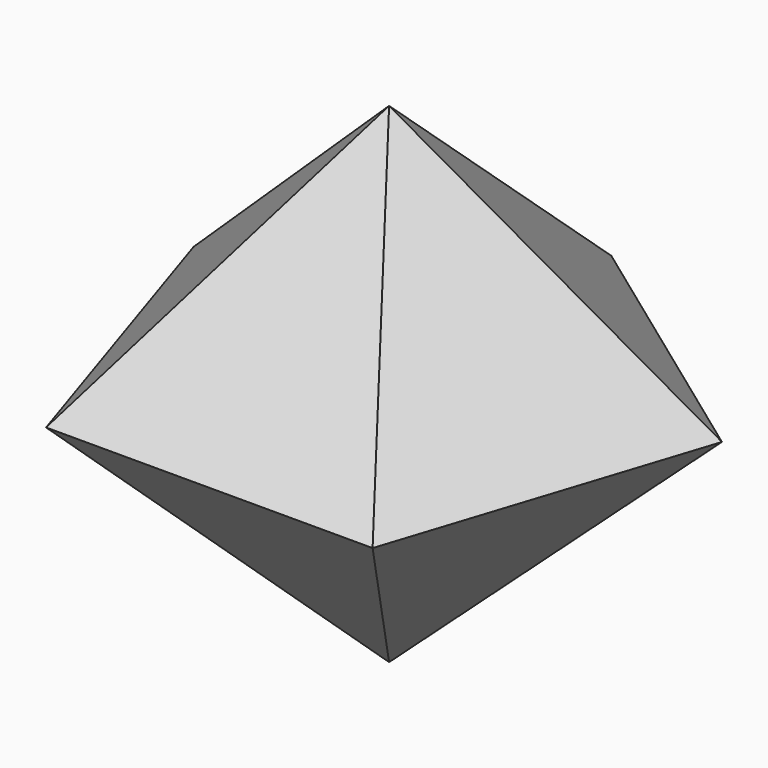
from build123d import *


with BuildPart() as f2:
    # F0 (on Top) → F2 section 0
    with BuildSketch(Plane.XY, mode=Mode.PRIVATE) as f2_s0:
        Polygon((12.7, -17.48005039), (20.5490316571, 6.6767851239), (0, 21.6065305321), (-20.5490316571, 6.6767851239), (-12.7, -17.48005039), align=None)
    loft([f2_s0.sketch, Vertex(0, 0, 19.05)])

    # F0 (on Top) → F3 section 0
    with BuildSketch(Plane.XY, mode=Mode.PRIVATE) as f3_s0:
        Polygon((12.7, -17.48005039), (20.5490316571, 6.6767851239), (0, 21.6065305321), (-20.5490316571, 6.6767851239), (-12.7, -17.48005039), align=None)
    loft([f3_s0.sketch, Vertex(0, 0, -19.05)])


solid = f2.part
